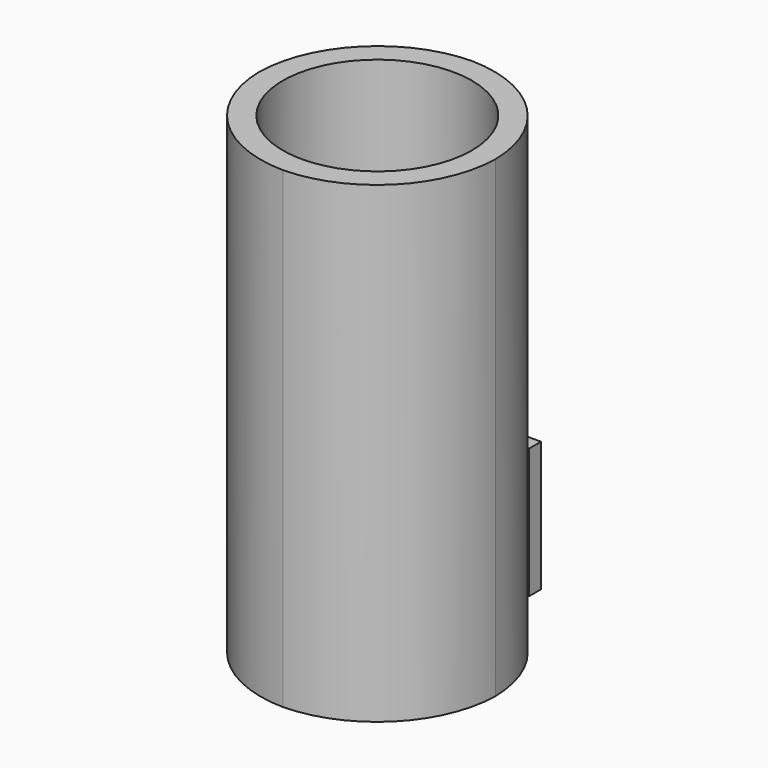
from build123d import *

# Parameters (mm, degrees)
F0_W          = 28
F0_H          = 55
F0_R          = 1.6
F1_DEPTH      = 6.35
F2_W          = 10
F2_H          = 40
F3_DEPTH      = 12.7
F4_W          = 100
F4_H          = 200
F5_DEPTH      = 100
F6_R          = 40
F7_DEPTH      = 177.8
F8_R          = 12.7
F9_DEPTH      = 41.656
F10_T1_DEPTH  = 454
F10_T6_DEPTH  = 454
F10_T12_DEPTH = 454
F10_T18_DEPTH = 454
F10_T25_DEPTH = 454
F10_T31_DEPTH = 454
F10_T37_DEPTH = 454
F10_T43_DEPTH = 454
F10_T49_DEPTH = 454
F10_T56_DEPTH = 454
F10_T62_DEPTH = 454


# Not quite as in the source:
# - a fillet or chamfer that OpenCascade refuses, or shapes differently, is made with other operations: its cross-section is extruded or revolved along the edge and cut away or added


with BuildPart() as f1:
    # F0 (on Front) → F1 (new body)
    with BuildSketch(Plane.XZ):
        Rectangle(F0_W, F0_H)
        with Locations((-9.5, -24)):
            Circle(F0_R, mode=Mode.SUBTRACT)
        with Locations((9.5, -24)):
            Circle(F0_R, mode=Mode.SUBTRACT)
        with Locations((-9.5, 0)):
            Circle(F0_R, mode=Mode.SUBTRACT)
        with Locations((-9.5, 24)):
            Circle(F0_R, mode=Mode.SUBTRACT)
        with Locations((9.5, 0)):
            Circle(F0_R, mode=Mode.SUBTRACT)
        with Locations((9.5, 24)):
            Circle(F0_R, mode=Mode.SUBTRACT)
    extrude(amount=F1_DEPTH)

    # F2 (on face) → F3 (join)
    with BuildSketch(Plane.XZ.offset(6.35)):
        Rectangle(F2_W, F2_H)
    extrude(amount=F3_DEPTH)

    # F4 (on face) → F5 (join)
    with BuildSketch(Plane.XZ.offset(19.05)):
        with Locations((0, 72.5)):
            Rectangle(F4_W, F4_H)
    extrude(amount=F5_DEPTH)

    # F6 (on face) → F7 (cut)
    with BuildSketch(Plane.XY.offset(172.5)):
        with Locations((0, -69.05)):
            Circle(F6_R)
    extrude(amount=-F7_DEPTH, mode=Mode.SUBTRACT)

    # F8 (on face) → F9 (cut)
    with BuildSketch(Plane.XY.offset(-5.3)):
        with Locations((0, -69.05)):
            Circle(F8_R)
    extrude(amount=-F9_DEPTH, mode=Mode.SUBTRACT)

    # F10: fillet of radius 50.8 on 4 edges, made by hand

    # F10_s2 → F10_t1 (cut)
    with BuildSketch(Plane.XY.offset(-154.5)):
        with BuildLine():
            ThreePointArc((-0.8, -119.05), (35.1210244843, -104.1710244843), (50, -68.25))
            Line((50, -68.25), (50, -119.05))
            Line((50, -119.05), (-0.8, -119.05))
        make_face()
        with BuildLine():
            ThreePointArc((-50, -68.25), (-35.1210244843, -104.1710244843), (0.8, -119.05))
            Line((0.8, -119.05), (-50, -119.05))
            Line((-50, -119.05), (-50, -68.25))
        make_face()
    extrude(amount=F10_T1_DEPTH, mode=Mode.SUBTRACT)


with BuildPart() as f10_tool4:
    # F10_s5 → F10_t6 (new body)
    with BuildSketch(Plane.XY.offset(-154.5)):
        with BuildLine():
            ThreePointArc((-0.8, -19.05), (35.1210244843, -33.9289755157), (50, -69.85))
            Line((50, -69.85), (50, -19.05))
            Line((50, -19.05), (-0.8, -19.05))
        make_face()
    extrude(amount=F10_T6_DEPTH)

    split(bisect_by=Plane.XY.offset(-20), keep=Keep.BOTTOM)

    split(bisect_by=Plane.YZ.offset(5), keep=Keep.BOTTOM)


with BuildPart() as f1_1:
    add(f1.part)

    # F10_t3: cut F10_tool4
    add(f10_tool4.part, mode=Mode.SUBTRACT)


with BuildPart() as f10_tool10:
    # F10_s11 → F10_t12 (new body)
    with BuildSketch(Plane.XY.offset(-154.5)):
        with BuildLine():
            ThreePointArc((-0.8, -19.05), (35.1210244843, -33.9289755157), (50, -69.85))
            Line((50, -69.85), (50, -19.05))
            Line((50, -19.05), (-0.8, -19.05))
        make_face()
    extrude(amount=F10_T12_DEPTH)

    split(bisect_by=Plane.XY.offset(-20), keep=Keep.BOTTOM)

    split(bisect_by=Plane.YZ.offset(5), keep=Keep.TOP)


with BuildPart() as f1_2:
    add(f1_1.part)

    # F10_t9: cut F10_tool10
    add(f10_tool10.part, mode=Mode.SUBTRACT)


with BuildPart() as f10_tool16:
    # F10_s17 → F10_t18 (new body)
    with BuildSketch(Plane.XY.offset(-154.5)):
        with BuildLine():
            ThreePointArc((-0.8, -19.05), (35.1210244843, -33.9289755157), (50, -69.85))
            Line((50, -69.85), (50, -19.05))
            Line((50, -19.05), (-0.8, -19.05))
        make_face()
    extrude(amount=F10_T18_DEPTH)

    split(bisect_by=Plane.XY.offset(20), keep=Keep.BOTTOM)

    split(bisect_by=Plane.XY.offset(-20), keep=Keep.TOP)

    split(bisect_by=Plane.YZ.offset(5), keep=Keep.TOP)


with BuildPart() as f1_3:
    add(f1_2.part)

    # F10_t15: cut F10_tool16
    add(f10_tool16.part, mode=Mode.SUBTRACT)


with BuildPart() as f10_tool23:
    # F10_s24 → F10_t25 (new body)
    with BuildSketch(Plane.XY.offset(-154.5)):
        with BuildLine():
            ThreePointArc((-0.8, -19.05), (35.1210244843, -33.9289755157), (50, -69.85))
            Line((50, -69.85), (50, -19.05))
            Line((50, -19.05), (-0.8, -19.05))
        make_face()
    extrude(amount=F10_T25_DEPTH)

    split(bisect_by=Plane.XY.offset(20), keep=Keep.TOP)

    split(bisect_by=Plane.YZ.offset(5), keep=Keep.BOTTOM)


with BuildPart() as f1_4:
    add(f1_3.part)

    # F10_t22: cut F10_tool23
    add(f10_tool23.part, mode=Mode.SUBTRACT)


with BuildPart() as f10_tool29:
    # F10_s30 → F10_t31 (new body)
    with BuildSketch(Plane.XY.offset(-154.5)):
        with BuildLine():
            ThreePointArc((-0.8, -19.05), (35.1210244843, -33.9289755157), (50, -69.85))
            Line((50, -69.85), (50, -19.05))
            Line((50, -19.05), (-0.8, -19.05))
        make_face()
    extrude(amount=F10_T31_DEPTH)

    split(bisect_by=Plane.XY.offset(20), keep=Keep.TOP)

    split(bisect_by=Plane.YZ.offset(5), keep=Keep.TOP)


with BuildPart() as f1_5:
    add(f1_4.part)

    # F10_t28: cut F10_tool29
    add(f10_tool29.part, mode=Mode.SUBTRACT)


with BuildPart() as f10_tool35:
    # F10_s36 → F10_t37 (new body)
    with BuildSketch(Plane.XY.offset(299.5)):
        with BuildLine():
            ThreePointArc((-50, -69.85), (-35.1210244843, -33.9289755157), (0.8, -19.05))
            Line((0.8, -19.05), (-50, -19.05))
            Line((-50, -19.05), (-50, -69.85))
        make_face()
    extrude(amount=-F10_T37_DEPTH)

    split(bisect_by=Plane.XY.offset(20), keep=Keep.TOP)

    split(bisect_by=Plane.YZ.offset(-5), keep=Keep.BOTTOM)


with BuildPart() as f1_6:
    add(f1_5.part)

    # F10_t34: cut F10_tool35
    add(f10_tool35.part, mode=Mode.SUBTRACT)


with BuildPart() as f10_tool41:
    # F10_s42 → F10_t43 (new body)
    with BuildSketch(Plane.XY.offset(299.5)):
        with BuildLine():
            ThreePointArc((-50, -69.85), (-35.1210244843, -33.9289755157), (0.8, -19.05))
            Line((0.8, -19.05), (-50, -19.05))
            Line((-50, -19.05), (-50, -69.85))
        make_face()
    extrude(amount=-F10_T43_DEPTH)

    split(bisect_by=Plane.XY.offset(20), keep=Keep.TOP)

    split(bisect_by=Plane.YZ.offset(-5), keep=Keep.TOP)


with BuildPart() as f1_7:
    add(f1_6.part)

    # F10_t40: cut F10_tool41
    add(f10_tool41.part, mode=Mode.SUBTRACT)


with BuildPart() as f10_tool47:
    # F10_s48 → F10_t49 (new body)
    with BuildSketch(Plane.XY.offset(299.5)):
        with BuildLine():
            ThreePointArc((-50, -69.85), (-35.1210244843, -33.9289755157), (0.8, -19.05))
            Line((0.8, -19.05), (-50, -19.05))
            Line((-50, -19.05), (-50, -69.85))
        make_face()
    extrude(amount=-F10_T49_DEPTH)

    split(bisect_by=Plane.XY.offset(20), keep=Keep.BOTTOM)

    split(bisect_by=Plane.YZ.offset(-5), keep=Keep.BOTTOM)

    split(bisect_by=Plane.XY.offset(-20), keep=Keep.TOP)


with BuildPart() as f1_8:
    add(f1_7.part)

    # F10_t46: cut F10_tool47
    add(f10_tool47.part, mode=Mode.SUBTRACT)


with BuildPart() as f10_tool54:
    # F10_s55 → F10_t56 (new body)
    with BuildSketch(Plane.XY.offset(299.5)):
        with BuildLine():
            ThreePointArc((-50, -69.85), (-35.1210244843, -33.9289755157), (0.8, -19.05))
            Line((0.8, -19.05), (-50, -19.05))
            Line((-50, -19.05), (-50, -69.85))
        make_face()
    extrude(amount=-F10_T56_DEPTH)

    split(bisect_by=Plane.YZ.offset(-5), keep=Keep.BOTTOM)

    split(bisect_by=Plane.XY.offset(-20), keep=Keep.BOTTOM)


with BuildPart() as f1_9:
    add(f1_8.part)

    # F10_t53: cut F10_tool54
    add(f10_tool54.part, mode=Mode.SUBTRACT)


with BuildPart() as f10_tool60:
    # F10_s61 → F10_t62 (new body)
    with BuildSketch(Plane.XY.offset(299.5)):
        with BuildLine():
            ThreePointArc((-50, -69.85), (-35.1210244843, -33.9289755157), (0.8, -19.05))
            Line((0.8, -19.05), (-50, -19.05))
            Line((-50, -19.05), (-50, -69.85))
        make_face()
    extrude(amount=-F10_T62_DEPTH)

    split(bisect_by=Plane.YZ.offset(-5), keep=Keep.TOP)

    split(bisect_by=Plane.XY.offset(-20), keep=Keep.BOTTOM)


with BuildPart() as f1_10:
    add(f1_9.part)

    # F10_t59: cut F10_tool60
    add(f10_tool60.part, mode=Mode.SUBTRACT)


solid = f1_10.part
